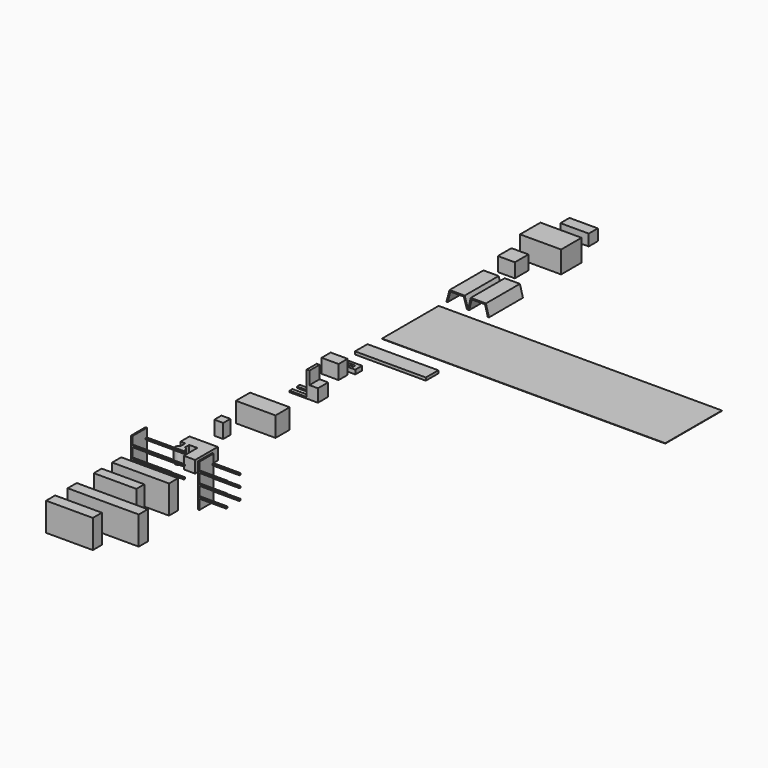
from build123d import *

# Parameters (mm, degrees)
F0_W      = 3300
F0_H      = 800
F1_DEPTH  = 2000
F0_W_2    = 5020
F2_DEPTH  = 2000
F0_W_3    = 3010
F0_H_2    = 700
F3_DEPTH  = 2000
F0_W_4    = 4010
F4_DEPTH  = 2000
F0_W_5    = 2800
F0_H_3    = 1260
F5_DEPTH  = 3000
F6_W      = 2700
F6_H      = 700
F7_DEPTH  = 1260
F8_W      = 2988.0481862915
F8_H      = 1060
F9_DEPTH  = 1700
F10_DEPTH = 850
F0_W_6    = 630
F0_H_4    = 630
F11_DEPTH = 1000
F0_H_5    = 1250
F12_DEPTH = 1400
F13_DEPTH = 1800
F14_W     = 1200
F14_H     = 1700
F14_W_2   = 603.0360460281
F14_H_2   = 900
F15_DEPTH = 900
F16_DEPTH = 300
F0_W_7    = 1200
F17_DEPTH = 1000
F0_W_8    = 5000
F0_H_6    = 1100
F18_DEPTH = 200
F0_W_9    = 20000
F0_H_7    = 5000
F19_DEPTH = 25
F0_W_10   = 3000
F0_H_8    = 3000
F20_DEPTH = 800
F22_DEPTH = 3000
F0_H_9    = 1200
F23_DEPTH = 1000
F25_W     = 800
F25_H     = 100
F26_DEPTH = 2700
F27_W     = 2900
F27_H     = 1800
F28_DEPTH = 1550
F0_W_11   = 2000
F29_DEPTH = 800


# Not quite as in the source:
# - a feature names something its author has since deleted; it is built from what else it names


with BuildPart() as f1:
    # F0 (on Top) → F1 (new body)
    with BuildSketch(Plane.XY):
        with Locations((1650, 400)):
            Rectangle(F0_W, F0_H)
    extrude(amount=F1_DEPTH)


with BuildPart() as f2:
    # F0 (on Top) → F2 (new body)
    with BuildSketch(Plane.XY):
        with Locations((2510, 2303.160572052)):
            Rectangle(F0_W_2, F0_H)
    extrude(amount=F2_DEPTH)


with BuildPart() as f3:
    # F0 (on Top) → F3 (new body)
    with BuildSketch(Plane.XY):
        with Locations((1505, 4557.8938484192)):
            Rectangle(F0_W_3, F0_H_2)
    extrude(amount=F3_DEPTH)


with BuildPart() as f4:
    # F0 (on Top) → F4 (new body)
    with BuildSketch(Plane.XY):
        with Locations((2005, 6236.0805511475)):
            Rectangle(F0_W_4, F0_H)
    extrude(amount=F4_DEPTH)


with BuildPart() as f5:
    # F0 (on Top) → F5 (new body)
    with BuildSketch(Plane.XY):
        with Locations((1400, 8139.4137191772)):
            Rectangle(F0_W_5, F0_H_3)
    extrude(amount=F5_DEPTH)

    # F6 (on face) → F7 (cut, through all)
    with BuildSketch(Plane(origin=(0, 8769.4137191772, 0), x_dir=(-1, 0, 0), z_dir=(0, 1, 0))):
        with Locations((-1450, 350)):
            Rectangle(F6_W, F6_H)
        with Locations((-1450, 1150)):
            Rectangle(F6_W, F6_H)
        with Locations((-1450, 1950)):
            Rectangle(F6_W, F6_H)
        with Locations((-1450, 2750)):
            Rectangle(F6_W, F6_H)
    extrude(amount=-F7_DEPTH, mode=Mode.SUBTRACT)

    # F8 (on face) → F9 (cut, through all)
    with BuildSketch(Plane.XY.offset(2400)):
        with Locations((1594.0240931458, 8139.4137191772)):
            Rectangle(F8_W, F8_H)
    extrude(amount=-F9_DEPTH, mode=Mode.SUBTRACT)


with BuildPart() as f10:
    # F0 (on Top) → F10 (new body)
    with BuildSketch(Plane.XY):
        with BuildLine():
            Line((0, 12653.9237976074), (0, 11853.9237976074))
            Line((0, 11853.9237976074), (342.5268346084, 11853.9237976074))
            Line((342.5268346084, 11853.9237976074), (342.5268346084, 11484.6496938236))
            ThreePointArc((342.5268346084, 11484.6496938236), (513.6710875982, 10838.0149080306), (624.5342638872, 11497.6634945311))
            Line((624.5342638872, 11497.6634945311), (624.5342638872, 11853.9237976074))
            Line((624.5342638872, 11853.9237976074), (1200, 11853.9237976074))
            Line((1200, 11853.9237976074), (1200, 10653.9237976074))
            Line((1200, 10653.9237976074), (2000, 10653.9237976074))
            Line((2000, 10653.9237976074), (2000, 12653.9237976074))
            Line((2000, 12653.9237976074), (0, 12653.9237976074))
        make_face()
    extrude(amount=F10_DEPTH)


with BuildPart() as f11:
    # F0 (on Top) → F11 (new body)
    with BuildSketch(Plane.XY):
        with Locations((315, 15161.4441299438)):
            Rectangle(F0_W_6, F0_H_4)
    extrude(amount=F11_DEPTH)


with BuildPart() as f12:
    # F0 (on Top) → F12 (new body)
    with BuildSketch(Plane.XY):
        with Locations((1400, 17373.9547729492)):
            Rectangle(F0_W_5, F0_H_5)
    extrude(amount=F12_DEPTH)


with BuildPart() as f13:
    # F0 (on Top) → F13 (new body)
    with BuildSketch(Plane.XY):
        Polygon((0, 21740.576171875), (0, 21490.576171875), (2000, 21490.576171875), (2000, 22390.576171875), (0, 22390.576171875), (0, 22140.576171875), (1200, 22140.576171875), (1200, 21740.576171875), align=None)
    extrude(amount=F13_DEPTH)

    # F14 (on face) → F15 (cut, through all)
    with BuildSketch(Plane.XZ.offset(-21490.576171875)):
        with Locations((600, 950)):
            Rectangle(F14_W, F14_H)
        with Locations((1698.4819769859, 1350)):
            Rectangle(F14_W_2, F14_H_2)
    extrude(amount=-F15_DEPTH, mode=Mode.SUBTRACT)


with BuildPart() as f16:
    # F0 (on Top) → F16 (new body)
    with BuildSketch(Plane.XY):
        Polygon((0, 25609.3289375305), (0, 25414.2469406128), (1500, 25414.2469406128), (1500, 26014.2469406128), (0, 26014.2469406128), (0, 25804.4109344482), (1200, 25804.4109344482), (1200, 25609.3289375305), align=None)
    extrude(amount=F16_DEPTH)


with BuildPart() as f17:
    # F0 (on Top) → F17 (new body)
    with BuildSketch(Plane.XY):
        with Locations((600, 24712.9100799561)):
            Rectangle(F0_W_7, F0_H)
    extrude(amount=F17_DEPTH)


with BuildPart() as f18:
    # F0 (on Top) → F18 (new body)
    with BuildSketch(Plane.XY):
        with Locations((2500, 27812.659072876)):
            Rectangle(F0_W_8, F0_H_6)
    extrude(amount=F18_DEPTH)


with BuildPart() as f19:
    # F0 (on Top) → F19 (new body)
    with BuildSketch(Plane.XY):
        with Locations((10000, 32144.1459655762)):
            Rectangle(F0_W_9, F0_H_7)
    extrude(amount=F19_DEPTH)


with BuildPart() as f20:
    # F0 (on Top) → F20 (new body)
    with BuildSketch(Plane.XY):
        with Locations((1500, 36835.0563049316)):
            Rectangle(F0_W_10, F0_H_8)
    extrude(amount=F20_DEPTH)

    # F21 (on face) → F22 (cut, through all)
    with BuildSketch(Plane.XZ.offset(-35335.0563049316)):
        Polygon((0, 800), (0, 0), (214.3593539449, 800), align=None)
        Polygon((1714.5810461517, 800), (1285.4189538483, 800), (1526.6357693569, 0), align=None)
        Polygon((3000, 800), (2785.6406460551, 800), (3000, 0), align=None)
        Polygon((275.7455129832, 720), (82.8220944328, 0), (1443.0782710648, 0), (1225.983137107, 720), align=None)
        Polygon((1777.9645828854, 720), (1608.8138337701, 0), (2917.1779055672, 0), (2724.2544870168, 720), align=None)
    extrude(amount=-F22_DEPTH, mode=Mode.SUBTRACT)


with BuildPart() as f23:
    # F0 (on Top) → F23 (new body)
    with BuildSketch(Plane.XY):
        with Locations((600, 40469.7204589844)):
            Rectangle(F0_W_7, F0_H_9)
    extrude(amount=F23_DEPTH)


with BuildPart() as f24_1:
    # F24: copy of F5
    add(f5.part.moved(Location((4800, -100, 0))))

    # F25 (on face) → F26 (cut)
    with BuildSketch(Plane.XY.offset(2400)):
        Polygon((9301.088013608, 9228.2405896963), (6800, 9228.2405896963), (6800, 7509.4137191772), (7600, 7509.4137191772), (7600, 7409.4137191772), (6800, 7409.4137191772), (6800, 6951.2433008371), (9301.088013608, 6951.2433008371), align=None)
        with Locations((7200, 7459.4137191772)):
            Rectangle(F25_W, F25_H)
    extrude(amount=-F26_DEPTH, mode=Mode.SUBTRACT)


with BuildPart() as f28:
    # F27 (on Top) → F28 (new body)
    with BuildSketch(Plane.XY):
        with Locations((1450, 42726.8852233887)):
            Rectangle(F27_W, F27_H)
    extrude(amount=F28_DEPTH)


with BuildPart() as f29:
    # F0 (on Top) → F29 (new body)
    with BuildSketch(Plane.XY):
        with Locations((1000, 45788.5299682617)):
            Rectangle(F0_W_11, F0_H)
    extrude(amount=F29_DEPTH)


solid = Compound([f1.part, f2.part, f3.part, f4.part, f5.part, f10.part, f11.part, f12.part, f13.part, f16.part, f17.part, f18.part, f19.part, f20.part, f23.part, f24_1.part, f28.part, f29.part])
